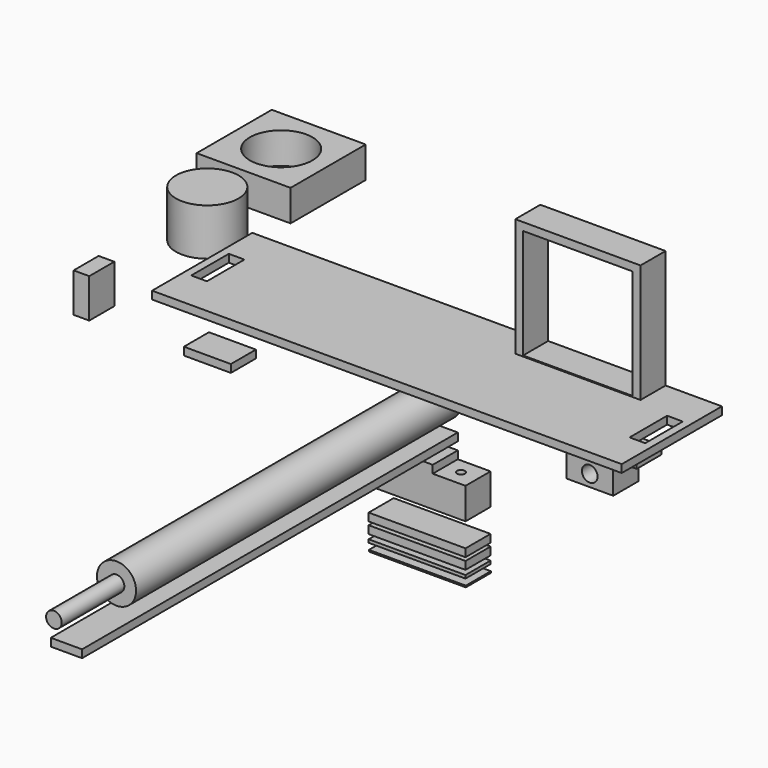
from build123d import *

# Parameters (mm, degrees)
F0_R      = 5
F1_DEPTH  = 20
F0_W      = 60
F0_H      = 5
F0_W_2    = 80
F0_H_2    = 80
F0_W_3    = 70
F0_H_3    = 70
F0_W_4    = 61.861140081
F0_H_4    = 1
F0_H_5    = 2
F0_R_2    = 12.5
F2_DEPTH  = 260
F3_R      = 5
F4_DEPTH  = 50
F5_DEPTH  = 300
F6_R      = 2.5
F7_R      = 2.5
F8_DEPTH  = 25
F10_R     = 2.5
F9_R      = 2.5
F11_DEPTH = 25
F16_R     = 5
F17_DEPTH = 50
F18_W     = 300
F18_H     = 5
F19_DEPTH = 80
F21_R     = 20
F22_DEPTH = 30
F21_W     = 60
F21_H     = 60
F23_DEPTH = 20
F20_W     = 10
F20_H     = 30
F24_DEPTH = 141.7069985357
F20_H_2   = 20
F25_DEPTH = 25
F20_W_2   = 30
F26_DEPTH = 5


# Not quite as in the source:
# - a feature of the source that left no trace in its solid (it failed there, or was rolled back) is left out
# - a feature names something its author has since deleted; it is built from what else it names


with BuildPart() as f1:
    # F0 (on Front) → F1 (new body)
    with BuildSketch(Plane.XZ):
        Polygon((95.2936565876, -7.5), (110.2936565876, -7.5), (125.2936565876, -7.5), (125.2936565876, 12.5), (140.2936565876, 12.5), (140.2936565876, 17.5), (110.2936565876, 17.5), (80.2936565876, 17.5), (80.2936565876, 12.5), (95.2936565876, 12.5), align=None)
        with Locations((110.2936565876, 0)):
            Circle(F0_R, mode=Mode.SUBTRACT)
    extrude(amount=F1_DEPTH)

    # F10 (on face) + F9 (on face) → F11 (cut)
    with BuildSketch(Plane(origin=(0, 0, 12.5), x_dir=(1, 0, 0), z_dir=(0, 0, -1))):
        with Locations((87.7936565876, 10)):
            Circle(F10_R)
    with BuildSketch(Plane(origin=(0, 0, 12.5), x_dir=(1, 0, 0), z_dir=(0, 0, -1))):
        with Locations((132.7936565876, 10)):
            Circle(F9_R)
    extrude(amount=-F11_DEPTH, mode=Mode.SUBTRACT)


with BuildPart() as f1b:
    # F0 (on Front) → F1, piece 2 (new body)
    with BuildSketch(Plane.XZ):
        with Locations((0, 29.2427036911)):
            Rectangle(F0_W, F0_H)
    extrude(amount=F1_DEPTH)


with BuildPart() as f1c:
    # F0 (on Front) → F1, piece 3 (new body)
    with BuildSketch(Plane.XZ):
        Polygon((10, -27.5771580637), (0, -27.5771580637), (-10, -27.5771580637), (-10, -32.5771580637), (-10.9305700405, -32.5771580637), (-30.9305700405, -32.5771580637), (-30.9305700405, -52.5771580637), (0, -52.5771580637), (30.9305700405, -52.5771580637), (30.9305700405, -32.5771580637), (10.9305700405, -32.5771580637), (10, -32.5771580637), align=None)
    extrude(amount=F1_DEPTH)

    # F6 (on face) + F7 (on face) → F8 (cut)
    with BuildSketch(Plane.XY.offset(-32.5771580637)):
        with Locations((-20, -10)):
            Circle(F6_R)
    with BuildSketch(Plane.XY.offset(-32.5771580637)):
        with Locations((20, -10)):
            Circle(F7_R)
    extrude(amount=-F8_DEPTH, mode=Mode.SUBTRACT)


with BuildPart() as f1d:
    # F0 (on Front) → F1, piece 4 (new body)
    with BuildSketch(Plane.XZ):
        with Locations((102.7326732874, 87.7068325877)):
            Rectangle(F0_W_2, F0_H_2)
        with Locations((102.7326732874, 87.7068325877)):
            Rectangle(F0_W_3, F0_H_3, mode=Mode.SUBTRACT)
    extrude(amount=F1_DEPTH)


with BuildPart() as f1e:
    # F0 (on Front) → F1, piece 5 (new body)
    with BuildSketch(Plane.XZ):
        with Locations((0, -77.355325222)):
            Rectangle(F0_W_4, F0_H)
    extrude(amount=F1_DEPTH)


with BuildPart() as f1f:
    # F0 (on Front) → F1, piece 6 (new body)
    with BuildSketch(Plane.XZ):
        with Locations((0.1928325291, -89.1451310813)):
            Rectangle(F0_W_4, F0_H_4)
    extrude(amount=F1_DEPTH)


with BuildPart() as f1g:
    # F0 (on Front) → F1, piece 7 (new body)
    with BuildSketch(Plane.XZ):
        with Locations((0, -83.756296128)):
            Rectangle(F0_W_4, F0_H_5)
    extrude(amount=F1_DEPTH)


with BuildPart() as f1h:
    # F0 (on Front) → F1, piece 8 (new body)
    with BuildSketch(Plane.XZ):
        with Locations((0, -70.2389810979)):
            Rectangle(F0_W_4, F0_H)
    extrude(amount=F1_DEPTH)


with BuildPart() as f2:
    # F0 (on Front) → F2 (new body)
    with BuildSketch(Plane.XZ):
        Circle(F0_R_2)
    extrude(amount=F2_DEPTH)

    # F3 (on face) → F4 (join)
    with BuildSketch(Plane.XZ.offset(260)):
        Circle(F3_R)
    extrude(amount=F4_DEPTH)

    # F16 (on face) → F17 (join)
    with BuildSketch(Plane(origin=(0, 0, 0), x_dir=(-1, 0, 0), z_dir=(0, 1, 0))):
        Circle(F16_R)
    extrude(amount=F17_DEPTH)


with BuildPart() as f5:
    # F0 (on Front) → F5 (new body)
    with BuildSketch(Plane.XZ):
        Polygon((-10, -22.5167013705), (0, -22.5167013705), (10, -22.5167013705), (10, -17.5167013705), (0, -17.5167013705), (-10, -17.5167013705), align=None)
    extrude(amount=F5_DEPTH)


with BuildPart() as f19:
    # F18 (on Front) → F19 (new body)
    with BuildSketch(Plane.XZ):
        with Locations((28.7307251245, 49.5608674544)):
            Rectangle(F18_W, F18_H)
    extrude(amount=F19_DEPTH)

    # F20 (on face) → F24 (cut, through all)
    with BuildSketch(Plane.XY.offset(52.0608674544)):
        with Locations((-111.2692748755, -40)):
            Rectangle(F20_W, F20_H)
        with Locations((168.7307251245, -40)):
            Rectangle(F20_W, F20_H)
    extrude(amount=-F24_DEPTH, mode=Mode.SUBTRACT)


with BuildPart() as f22:
    # F21 (on Top) → F22 (new body)
    with BuildSketch(Plane.XY):
        with Locations((-196.2528675795, 57.794149965)):
            Circle(F21_R)
    extrude(amount=F22_DEPTH)


with BuildPart() as f23:
    # F21 (on Top) → F23 (new body)
    with BuildSketch(Plane.XY):
        with Locations((-205.1943850517, 127.9719012976)):
            Rectangle(F21_W, F21_H)
        with Locations((-205.1943850517, 127.9719012976)):
            Circle(F21_R, mode=Mode.SUBTRACT)
    extrude(amount=F23_DEPTH)


with BuildPart() as f25:
    # F20 (on face) → F25 (new body)
    with BuildSketch(Plane.XY.offset(52.0608674544)):
        with Locations((-130.5344802141, -114.8494374752)):
            Rectangle(F20_W, F20_H_2)
    extrude(amount=F25_DEPTH)


with BuildPart() as f26:
    # F20 (on face) → F26 (new body)
    with BuildSketch(Plane.XY.offset(52.0608674544)):
        with Locations((-50.0688782334, -114.8494374752)):
            Rectangle(F20_W_2, F20_H_2)
    extrude(amount=F26_DEPTH)


solid = Compound([f1.part, f1b.part, f1c.part, f1d.part, f1e.part, f1f.part, f1g.part, f1h.part, f2.part, f5.part, f19.part, f22.part, f23.part, f25.part, f26.part])
